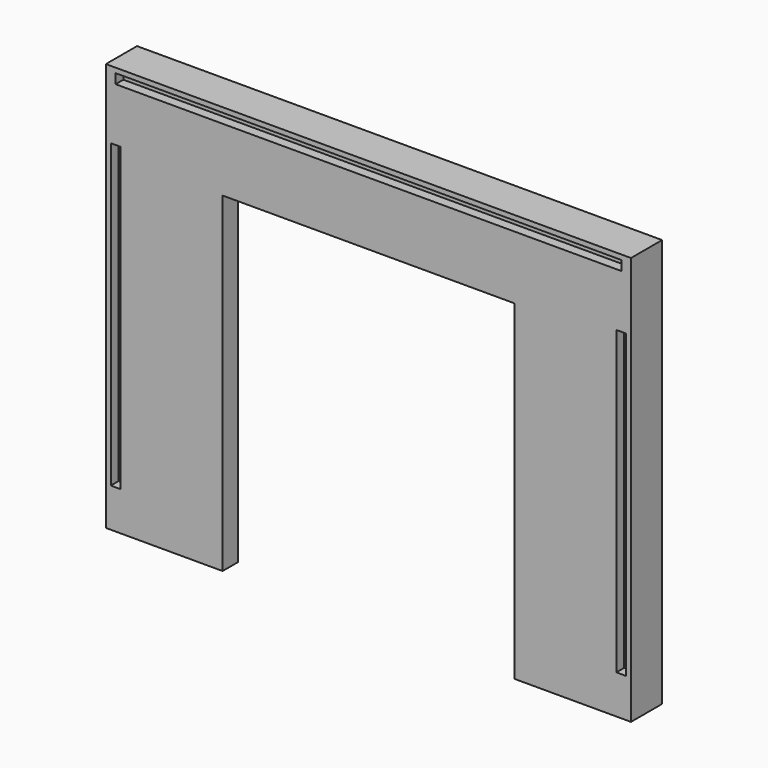
from build123d import *

# Parameters (mm, degrees)
F0_W      = 342.9
F0_H      = 266.7
F1_DEPTH  = 25.4
F2_W      = 114.3
F2_H      = 215.9
F3_DEPTH  = 25.4
F4_W      = 12.7
F4_H      = 215.9
F5_DEPTH  = 19.05
F6_W      = 12.7
F6_H      = 215.9
F7_DEPTH  = 19.05
F9_W      = 330.2
F9_H      = 6.35
F10_DEPTH = 6.35
F11_W     = 6.35
F11_H     = 196.85
F12_DEPTH = 6.35


# Not quite as in the source:
# - a feature names something its author has since deleted; it is built from what else it names


with BuildPart() as f1:
    # F0 (on Front) → F1 (new body)
    with BuildSketch(Plane.XZ):
        with Locations((-171.45, 133.35)):
            Rectangle(F0_W, F0_H)
    extrude(amount=F1_DEPTH)

    # F2 (on face) → F3 (cut)
    with BuildSketch(Plane(origin=(0, 0, 0), x_dir=(-1, 0, 0), z_dir=(0, 1, 0))):
        with Locations((228.6, 107.95)):
            Rectangle(F2_W, F2_H)
        with Locations((114.3, 107.95)):
            Rectangle(F2_W, F2_H)
    extrude(amount=-F3_DEPTH, mode=Mode.SUBTRACT)

    # F4 (on face) → F5 (join)
    with BuildSketch(Plane.YZ.offset(-285.75)):
        with Locations((-19.05, 107.95)):
            Rectangle(F4_W, F4_H)
    extrude(amount=F5_DEPTH)

    # F6 (on face) → F7 (join)
    with BuildSketch(Plane(origin=(-57.15, 0, 0), x_dir=(0, -1, 0), z_dir=(-1, 0, 0))):
        with Locations((19.05, 107.95)):
            Rectangle(F6_W, F6_H)
    extrude(amount=F7_DEPTH)

    # F9 (on face) → F10 (cut)
    with BuildSketch(Plane.XZ.offset(25.4)):
        with Locations((-171.45, 260.35)):
            Rectangle(F9_W, F9_H)
    extrude(amount=-F10_DEPTH, mode=Mode.SUBTRACT)

    # F11 (on face) → F12 (cut)
    with BuildSketch(Plane.XZ.offset(25.4)):
        with Locations((-336.55, 123.825)):
            Rectangle(F11_W, F11_H)
        with Locations((-6.35, 123.825)):
            Rectangle(F11_W, F11_H)
    extrude(amount=-F12_DEPTH, mode=Mode.SUBTRACT)


solid = f1.part
